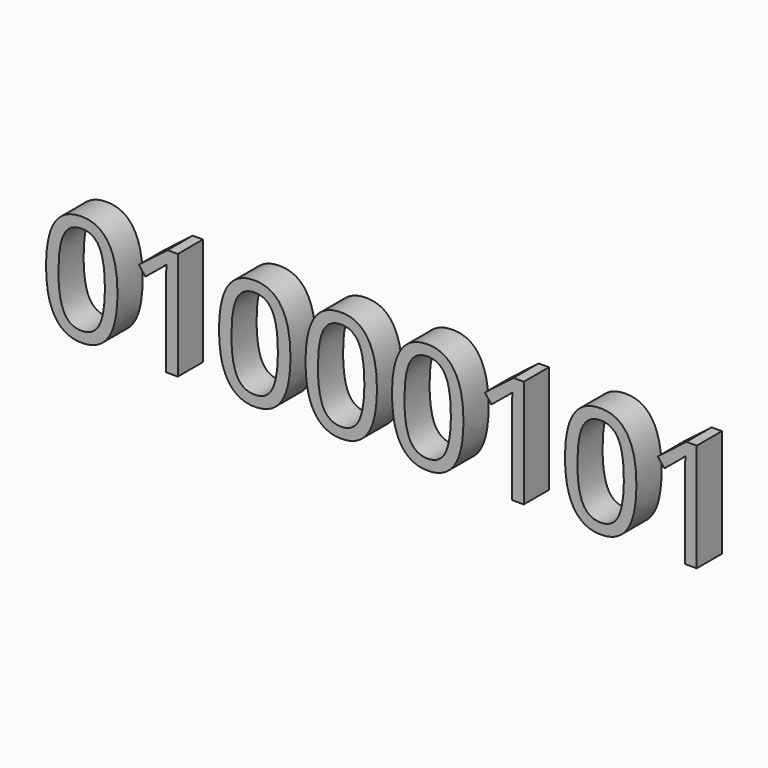
from build123d import *

# Parameters (mm, degrees)
F0_TEXT_SIZE = 122.1088640806
F1_DEPTH     = 25.4


# Not quite as in the source:
# - Text() gives the source's letters only with a copy of the font that has no kerning and outlines rounded to 1/6400 em; it was checked with that copy


with BuildPart() as f1:
    # F0 (on Front) → F1 (new body)
    with BuildSketch(Plane.XZ):
        with Locations((-76.6925513744, -31.7814610898)):
            Text('01000101', F0_TEXT_SIZE, font='Open Sans', text_align=(TextAlign.LEFT, TextAlign.BOTTOM))
    extrude(amount=F1_DEPTH)


solid = f1.part
